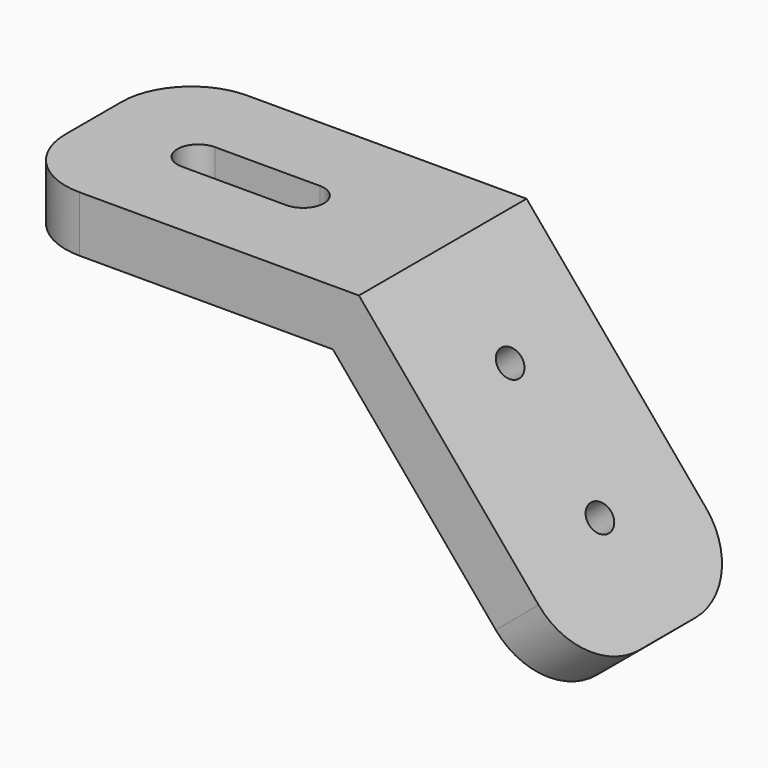
from build123d import *

# Parameters (mm, degrees)
F1_DEPTH = 15
F3_DEPTH = 43.4455230334
F5_D     = 4
F6_R     = 10


with BuildPart() as f1:
    # F0 (on Front) → F1 (new body, symmetric)
    with BuildSketch(Plane.XZ):
        Polygon((0, 8), (0, 0), (46.2695387348, 0), (76.0110249394, -35.4445230334), (82.1393804843, -30.3022221559), (50, 8), align=None)
    extrude(amount=F1_DEPTH, both=True)

    # F2 (on face) → F3 (cut, through all)
    with BuildSketch(Plane.XY.offset(8)):
        with BuildLine():
            ThreePointArc((15, 3), (12, 0), (15, -3))
            Line((15, -3), (30, -3))
            ThreePointArc((30, -3), (33, 0), (30, 3))
            Line((30, 3), (15, 3))
        make_face()
    extrude(amount=-F3_DEPTH, mode=Mode.SUBTRACT)

    # F5 (through all)
    with Locations(Plane(origin=(33.2804354537, 0, 27.9256011146), x_dir=(0, 1, 0), z_dir=(0.7660444431, 0, 0.6427876097))):
        with Locations((0, -41.0110249394), (0, -61.0110249394)):
            Hole(F5_D / 2)

    # F6
    f6_edges = [f1.edges().sort_by_distance(p)[0] for p in [
        (79.075203, -15, -32.873373),
        (79.075203, 15, -32.873373),
        (0, -15, 4),
        (0, 15, 4),
    ]]
    fillet(f6_edges, radius=F6_R)


solid = f1.part
